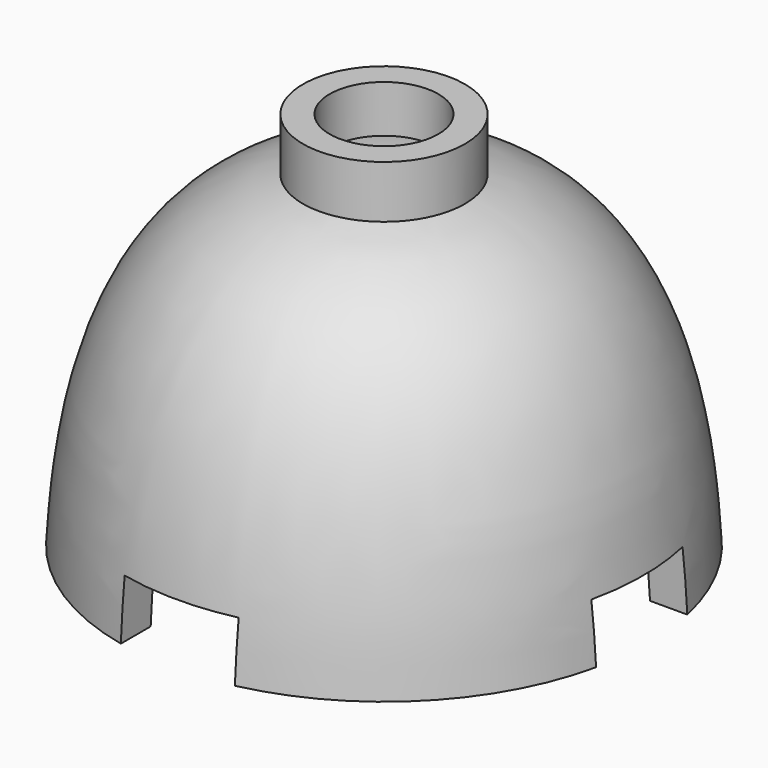
from build123d import *

# Parameters (mm, degrees)
F5_W      = 3.4
F5_H      = 1.75
F6_DEPTH  = 15.7710001
F8_W      = 3.4
F8_H      = 1.75
F9_DEPTH  = 15.7710001
F3_R      = 2.415
F3_R_2    = 1.62
F10_DEPTH = 11.4


# Not quite as in the source:
# - the dataset's text gives a spline's control points without its knots; the knots are read off the source's solid


with BuildPart() as f1:
    # F0 (on Right) → F1 (revolve)
    with BuildSketch(Plane.YZ):
        with BuildLine():
            add(Edge.make_bspline(
                [(0, 10.0184451824), (6.8137775206, 10.2505443388), (7.6669137151, 3.8190624776), (7.87, 0.0184451824)],
                knots=[0, 0, 0, 0, 12.7254430178, 12.7254430178, 12.7254430178, 12.7254430178], degree=3))
            Line((0, 10.0184451824), (0, 0.0184451824))
            Line((0, 0.0184451824), (0.0367669511, 8.9390710533))
            add(Edge.make_bspline(
                [(0.0367669511, 8.9390710533), (0.8033031519, 8.9651817393), (2.1235558491, 8.828403274), (3.5770824697, 8.2170500598), (4.6691932617, 7.288309401), (5.4993568364, 6.0632667187), (6.0939655872, 4.6044346653), (6.6030130693, 2.5101767004), (6.7383162854, 0.9310906536), (6.7884172037, 0.0184451824)],
                knots=[0, 0, 0, 0, 0.125, 0.25, 0.375, 0.5, 0.625, 0.75, 0.9948308485, 0.9948308485, 0.9948308485, 0.9948308485], degree=3))
            Line((6.7884172037, 0.0184451824), (7.87, 0.0184451824))
        make_face()
    revolve(axis=Axis((0, 0, 5.0184451824), (0, 0, -1)))

    # F5 (on offset) → F6 (cut, through all)
    with BuildSketch(Plane.XZ.offset(-7.9)):
        with Locations((0, 0.875)):
            Rectangle(F5_W, F5_H)
    extrude(amount=F6_DEPTH, mode=Mode.SUBTRACT)

    # F8 (on offset) → F9 (cut, through all)
    with BuildSketch(Plane.YZ.offset(7.9)):
        with Locations((0, 0.875)):
            Rectangle(F8_W, F8_H)
    extrude(amount=-F9_DEPTH, mode=Mode.SUBTRACT)

    # F3 (on offset) → F10 (join)
    with BuildSketch(Plane.XY.offset(11.35)):
        Circle(F3_R)
        Circle(F3_R_2, mode=Mode.SUBTRACT)
    extrude(amount=-F10_DEPTH)


solid = f1.part
